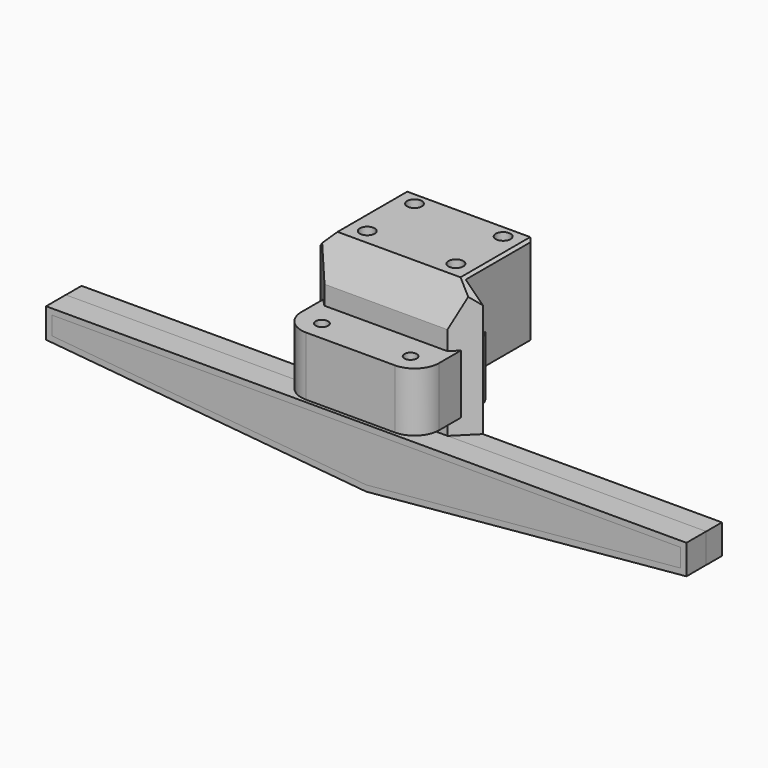
from build123d import *

# Parameters (mm, degrees)
F0_R         = 1.25
F1_DEPTH     = 12
F2_W         = 34.9669195712
F2_H         = 27
F2_H_2       = 8
F3_DEPTH     = 1
F4_DEPTH     = 20
F5_R         = 1.15
F6_DEPTH     = 3
F7_DEPTH     = 4
F8_DEPTH     = 10
F9_W         = 8
F9_H         = 17
F9_H_2       = 3
F10_DEPTH    = 17
F11_R        = 1.5
F12_DEPTH    = 18
F14_DEPTH    = 5
F15_T        = -1.2
F16_DEPTH    = 3.8
F19_SIZE     = 5
F20_SIZE     = 16.99999
F21_SIZE     = 3
F22_T1_DEPTH = 50.8936235002
F23_DEPTH    = 35


# Not quite as in the source:
# - a fillet or chamfer that OpenCascade refuses, or shapes differently, is made with other operations: its cross-section is extruded or revolved along the edge and cut away or added
# - a fillet or chamfer is up to 0.001 mm smaller than in the source, because OpenCascade refuses the exact size


with BuildPart() as f1:
    # F0 (on Top) → F1 (new body)
    with BuildSketch(Plane.XY):
        with BuildLine():
            ThreePointArc((14, 5), (12.5355339059, 8.5355339059), (9, 10))
            Line((9, 10), (-9, 10))
            ThreePointArc((-9, 10), (-12.5355339059, 8.5355339059), (-14, 5))
            Line((-14, 5), (-14, -5))
            ThreePointArc((-14, -5), (-12.5355339059, -8.5355339059), (-9, -10))
            Line((-9, -10), (9, -10))
            ThreePointArc((9, -10), (12.5355339059, -8.5355339059), (14, -5))
            Line((14, -5), (14, 5))
        make_face()
        with Locations((-9, -6)):
            Circle(F0_R, mode=Mode.SUBTRACT)
        with Locations((9, -6)):
            Circle(F0_R, mode=Mode.SUBTRACT)
        with Locations((-9, 6)):
            Circle(F0_R, mode=Mode.SUBTRACT)
        with Locations((9, 6)):
            Circle(F0_R, mode=Mode.SUBTRACT)
    extrude(amount=F1_DEPTH)


with BuildPart() as f3:
    # F2 (on Front) → F3 (new body)
    with BuildSketch(Plane.XZ):
        Polygon((-17.4834597856, -3.1417060565), (-65, -3.1417060565), (-65, -9.1417060565), (0, -15.1417060565), (65, -9.1417060565), (65, -3.1417060565), (17.4834597856, -3.1417060565), (17.4834597856, -11.1417060565), (-17.4834597856, -11.1417060565), align=None)
        with Locations((0, 10.3582939435)):
            Rectangle(F2_W, F2_H)
        with Locations((0, -7.1417060565)):
            Rectangle(F2_W, F2_H_2)
    extrude(amount=F3_DEPTH)

    # F2 (on Front) → F4 (join)
    with BuildSketch(Plane.XZ):
        with Locations((0, 10.3582939435)):
            Rectangle(F2_W, F2_H)
        with Locations((0, -7.1417060565)):
            Rectangle(F2_W, F2_H_2)
    extrude(amount=-F4_DEPTH)

    # F5 (on face) + F2 (on Front) → F6 (join)
    with BuildSketch(Plane.XZ.offset(1)):
        Polygon((-55, -10.0647829795), (-55, -3.1417060565), (-65, -3.1417060565), (-65, -9.1417060565), align=None)
        with Locations((-60, -6.1417060565)):
            Circle(F5_R, mode=Mode.SUBTRACT)
        Polygon((55, -3.1417060565), (55, -10.0647829795), (65, -9.1417060565), (65, -3.1417060565), align=None)
        with Locations((60, -6.1417060565)):
            Circle(F5_R, mode=Mode.SUBTRACT)
    with BuildSketch(Plane.XZ):
        Polygon((-17.4834597856, -3.1417060565), (-65, -3.1417060565), (-65, -9.1417060565), (0, -15.1417060565), (65, -9.1417060565), (65, -3.1417060565), (17.4834597856, -3.1417060565), (17.4834597856, -11.1417060565), (-17.4834597856, -11.1417060565), align=None)
    extrude(amount=-F6_DEPTH)

    # F5 (on face) → F7 (cut, through all)
    with BuildSketch(Plane.XZ.offset(1)):
        with Locations((-60, -6.1417060565)):
            Circle(F5_R)
        with Locations((60, -6.1417060565)):
            Circle(F5_R)
    extrude(amount=-F7_DEPTH, mode=Mode.SUBTRACT)

    # F5 (on face) → F8 (cut)
    with BuildSketch(Plane.XZ.offset(1)):
        with Locations((-14, -6.1417060565)):
            Circle(F5_R)
        with Locations((14, -6.1417060565)):
            Circle(F5_R)
    extrude(amount=-F8_DEPTH, mode=Mode.SUBTRACT)

    # F9 (on face) → F10 (cut)
    with BuildSketch(Plane(origin=(0, 0, -11.1417060565), x_dir=(1, 0, 0), z_dir=(0, 0, -1))):
        with Locations((9, -11.5)):
            Rectangle(F9_W, F9_H)
        with Locations((9, -1.5)):
            Rectangle(F9_W, F9_H_2)
        with Locations((-9, -11.5)):
            Rectangle(F9_W, F9_H)
        with Locations((-9, -1.5)):
            Rectangle(F9_W, F9_H_2)
    extrude(amount=-F10_DEPTH, mode=Mode.SUBTRACT)

    # F11 (on face) → F12 (cut, through all)
    with BuildSketch(Plane(origin=(0, 0, 5.8582939435), x_dir=(1, 0, 0), z_dir=(0, 0, -1))):
        with Locations((-9, -5.4900380783)):
            Circle(F11_R)
        with Locations((-9, -17.4900380783)):
            Circle(F11_R)
        with Locations((9, -5.4900380783)):
            Circle(F11_R)
        with Locations((9, -17.4900380783)):
            Circle(F11_R)
    extrude(amount=-F12_DEPTH, mode=Mode.SUBTRACT)

    # F19
    f19_edges = [f3.edges().sort_by_distance(p)[0] for p in [
        (-17.48346, -1, 10.358294),
        (17.48346, -1, 10.358294),
        (-17.48346, 20, 6.358294),
        (17.48346, 20, 6.358294),
        (-17.48346, 9.5, 23.858294),
        (17.48346, 9.5, 23.858294),
    ]]
    chamfer(f19_edges, length=F19_SIZE)

    # F20 (size 17 in the source; OpenCascade refuses exactly that, so slightly less here)
    f20_edges = [f3.edges().sort_by_distance(p)[0] for p in [
        (0, 20, -11.141706),
    ]]
    chamfer(f20_edges, length=F20_SIZE)

    # F21
    f21_edges = [f3.edges().sort_by_distance(p)[0] for p in [
        (0, -1, 23.858294),
    ]]
    chamfer(f21_edges, length=F21_SIZE)

    # F22: chamfer of 5 on 1 edges, made by hand

    # F22_s2 → F22_t1 (cut)
    with BuildSketch(Plane.YZ.offset(-25.4468117501)):
        Polygon((-1, 15.8582939435), (2.5355339059, 24.3938278495), (-1, 20.8582939435), align=None)
    extrude(amount=F22_T1_DEPTH, mode=Mode.SUBTRACT)

    # F23 (cut, through all): faces of the model
    f23_faces = [f3.faces().sort_by_distance(p)[0] for p in [
        (15.1081194146, 10.2337090854, -11.1417060565),
        (-15.1081194146, 10.2337090854, -11.1417060565),
    ]]
    extrude(f23_faces, amount=-F23_DEPTH, mode=Mode.SUBTRACT)


with BuildPart() as f14:
    # F13 (on face) → F14 (new body)
    with BuildSketch(Plane.XZ.offset(1)):
        Polygon((65, -2.4325364381), (-65, -2.4325364381), (-65, -8.4325364381), (0, -14.4325364381), (65, -8.4325364381), align=None)
    extrude(amount=F14_DEPTH)

    # F15
    f15_openings = [f14.faces().sort_by_distance(p)[0] for p in [
        (0, -6, -7.099203),
    ]]
    offset(amount=F15_T, openings=f15_openings)


with BuildPart() as f16:
    # F16 (new): a face of the model
    f16_faces = [f14.part.faces().sort_by_distance(p)[0] for p in [
        (0, -2.2, -7.1749809809),
    ]]
    extrude(f16_faces, amount=F16_DEPTH)


with BuildPart() as f14_1:
    # F17: moved
    add(f14.part.moved(Location((0, 0, -0.7))))


with BuildPart() as f16_1:
    # F18: moved
    add(f16.part.moved(Location((0, 0, -0.7))))


solid = Compound([f1.part, f3.part, f14_1.part, f16_1.part])
